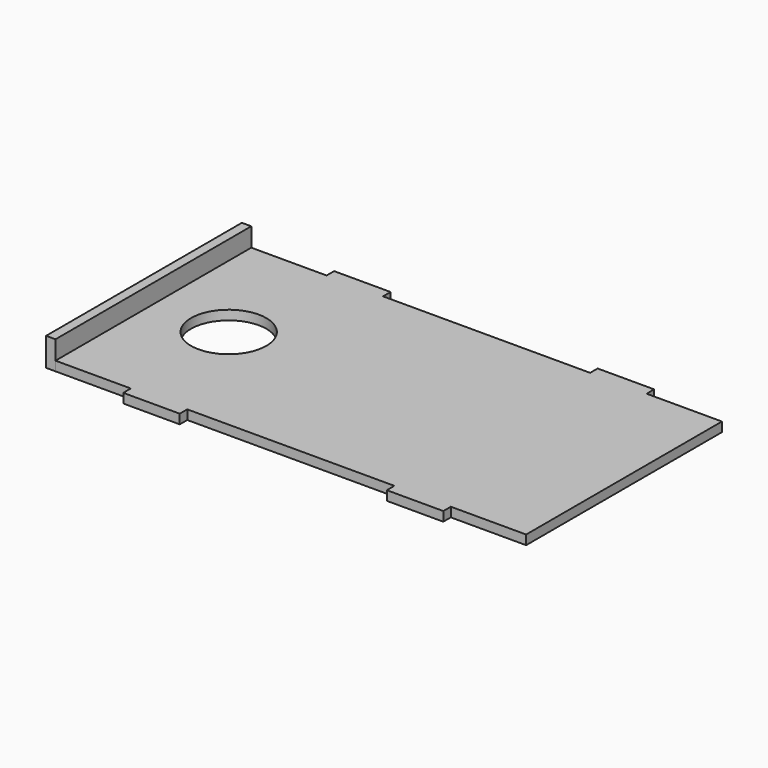
from build123d import *

# Parameters (mm, degrees)
F1_R     = 12.7
F2_DEPTH = 3.175
F3_W     = 31.75
F3_H     = 3.175
F4_DEPTH = 3.175


# Not quite as in the source:
# - a variable given as a bare number and used for a length is read in inches; the dataset says mm whatever the document's units were


with BuildPart() as f2:
    # F1 (on Top) → F2 (new body)
    with BuildSketch(Plane.XY):
        Polygon((-53.975, 41.275), (-79.375, 41.275), (-79.375, 9.525), (-82.55, 9.525), (-82.55, 0), (-82.55, -9.525), (-79.375, -9.525), (-79.375, -41.275), (-53.975, -41.275), (-53.975, -44.45), (-34.925, -44.45), (-34.925, -41.275), (34.925, -41.275), (34.925, -44.45), (53.975, -44.45), (53.975, -41.275), (79.375, -41.275), (79.375, 41.275), (53.975, 41.275), (53.975, 44.45), (34.925, 44.45), (34.925, 41.275), (-34.925, 41.275), (-34.925, 44.45), (-53.975, 44.45), align=None)
        with Locations((-53.975, 0)):
            Circle(F1_R, mode=Mode.SUBTRACT)
    extrude(amount=F2_DEPTH)


with BuildPart() as f4:
    # F3 (on face) → F4 (new body)
    with BuildSketch(Plane(origin=(-79.375, 0, 0), x_dir=(0, -1, 0), z_dir=(-1, 0, 0))):
        Polygon((-41.275, 9.525), (-41.275, 3.175), (-9.525, 3.175), (9.525, 3.175), (9.525, 0), (41.275, 0), (41.275, 9.525), align=None)
        with Locations((-25.4, 1.5875)):
            Rectangle(F3_W, F3_H)
    extrude(amount=F4_DEPTH)


solid = Compound([f2.part, f4.part])
